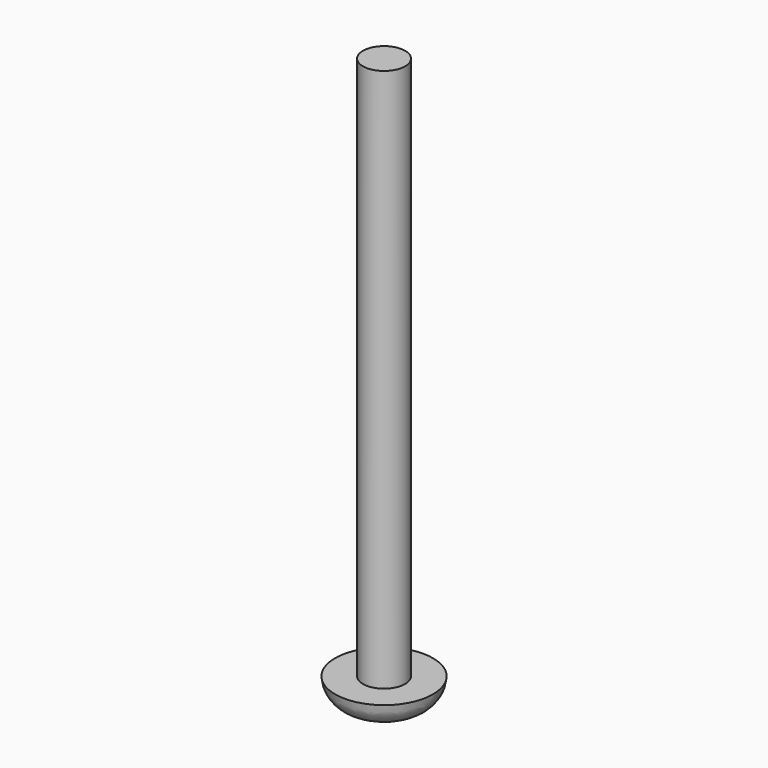
from build123d import *

# Parameters (mm, degrees)
F0_R          = 3.937
F1_DEPTH      = 101.6
F1_DEPTH_BACK = 2.54
F0_R_2        = 9.144
F2_DEPTH      = 4.7625


# Not quite as in the source:
# - a fillet or chamfer that OpenCascade refuses, or shapes differently, is made with other operations: its cross-section is extruded or revolved along the edge and cut away or added


with BuildPart() as f1:
    # F0 (on Top) → F1 (new body, two sides)
    with BuildSketch(Plane.XY) as f1_sk:
        Circle(F0_R)
    extrude(amount=F1_DEPTH)
    extrude(f1_sk.sketch, amount=-F1_DEPTH_BACK)

    # F0 (on Top) → F2 (join)
    with BuildSketch(Plane.XY):
        Circle(F0_R_2)
        Circle(F0_R, mode=Mode.SUBTRACT)
        Circle(F0_R)
    extrude(amount=-F2_DEPTH)

    # F3: fillet of radius 5.08 on 1 edges, made by hand

    # F3_s1 → F3_t2 (revolve, cut)
    with BuildSketch(Plane.XZ):
        with BuildLine():
            ThreePointArc((9.144, 0), (7.5519698235, -3.3851544532), (4.0739315833, -4.7625))
            Line((4.0739315833, -4.7625), (9.144, -4.7625))
            Line((9.144, -4.7625), (9.144, 0))
        make_face()
    revolve(axis=Axis((0, 0, -4.7625), (0, 0, 1)), mode=Mode.SUBTRACT)


solid = f1.part
